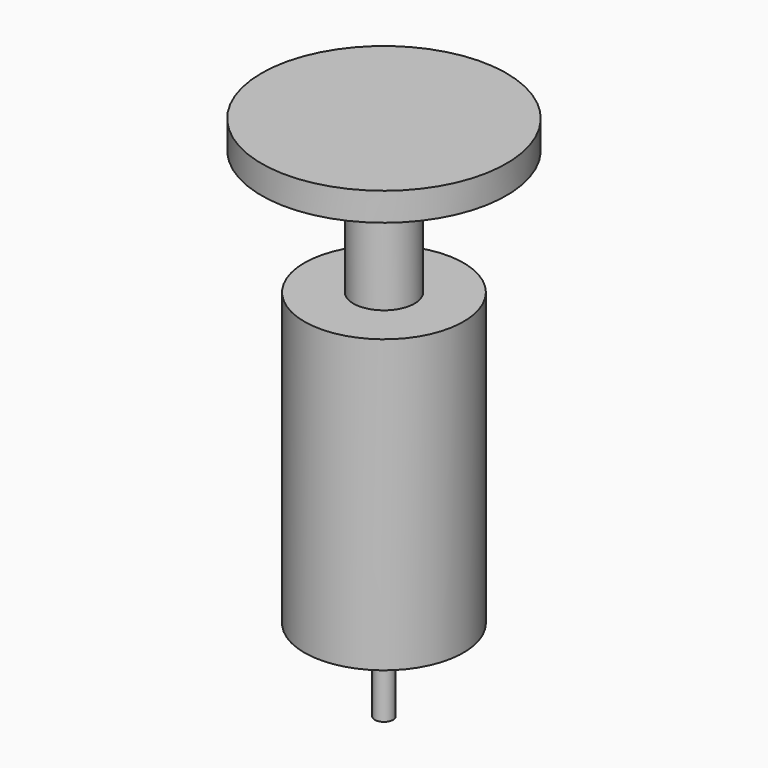
from build123d import *

# Parameters (mm, degrees)
F0_W = 2.4999999441
F0_H = 10.1996297166


# Not quite as in the source:
# - ends of sketch curves that miss each other by under 0.0002 mm in the source are joined


with BuildPart() as f1:
    # F0 (on Front) → F1 (revolve)
    with BuildSketch(Plane.XZ):
        Polygon((0, -34.0000009239), (0, -10.1996297166), (-2.4999999441, -10.1996297166), (-6.5000001341, -10.1996297166), (-6.5000001341, -34), (-0.75, -34), align=None)
        with Locations((-1.2499999721, -5.0998148583)):
            Rectangle(F0_W, F0_H)
        Polygon((0, 2.3), (-10, 2.3), (-10, 0), (-2.4999999441, 0), (0, 0), align=None)
        Polygon((0, -40.7000018477), (0, -34.0000009239), (-0.75, -34), (-0.75, -40.7000018477), align=None)
    revolve(axis=Axis((0, 0, -22.5782128982), (0, 0, -1)))


solid = f1.part
